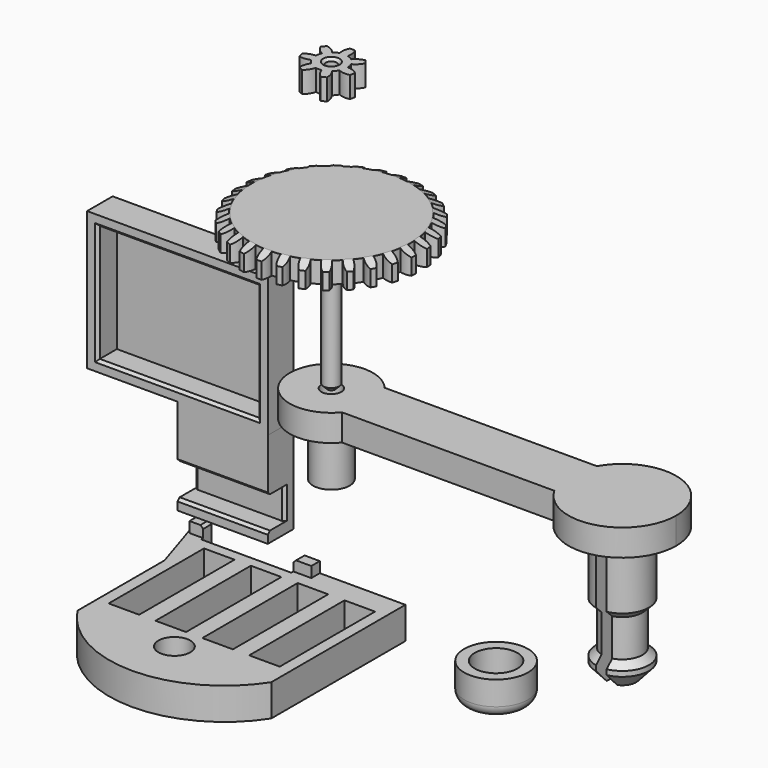
from build123d import *

# Parameters (mm, degrees)
F2_DEPTH   = 4
F3_R       = 1.05
F4_DEPTH   = 25
F5_SIZE    = 0.5
F7_DEPTH   = 4
F8_R       = 1.5
F9_DEPTH   = 25
F10_SIZE   = 0.8
F12_W      = 30
F12_H      = 22
F13_DEPTH  = 1.5
F12_W_2    = 16.9512806386
F12_H_2    = 18
F14_DEPTH  = 6
F16_W      = 5.7375021279
F16_H      = 22.3875014344
F16_R      = 3
F16_W_2    = 19.4487193614
F16_H_2    = 2
F17_DEPTH  = 6
F19_W      = 5.8088458058
F19_H      = 6
F20_DEPTH  = 25
F21_W      = 3.3711902797
F21_H      = 2
F22_DEPTH  = 2
F23_SIZE   = 0.5
F23_2_SIZE = 0.5
F26_DEPTH  = 5
F27_R      = 3.4403136116
F28_DEPTH  = 10
F29_R      = 1.35
F30_DEPTH  = 15
F30_TAPER  = -2
F31_R      = 5
F32_DEPTH  = 25
F33_W      = 2
F33_H      = 11.0666673959
F34_DEPTH  = 25
F38_R      = 6
F38_R_2    = 4
F39_DEPTH  = 6.5
F40_R      = 1.99999


# Not quite as in the source:
# - a fillet or chamfer is up to 0.001 mm smaller than in the source, because OpenCascade refuses the exact size


with BuildPart() as f2:
    # F1 (on offset) → F2 (new body)
    with BuildSketch(Plane.XY.offset(25)):
        with BuildLine():
            ThreePointArc((0.7727213217, 2.898775907), (0.8079351244, 3.9593943014), (0.5, 4.9749371855))
            ThreePointArc((0.5, 4.9749371855), (0, 5), (-0.5, 4.9749371855))
            ThreePointArc((-0.5, 4.9749371855), (-0.8079351244, 3.9593943014), (-0.7727213217, 2.898775907))
            ThreePointArc((-0.7727213217, 2.898775907), (-1.3029249894, 2.7055516185), (-1.7845704009, 2.4114950724))
            ThreePointArc((-1.7845704009, 2.4114950724), (-2.5918398057, 3.1003110845), (-3.577817614, 3.4927383413))
            ThreePointArc((-3.577817614, 3.4927383413), (-3.9091574123, 3.1174490093), (-4.2013074159, 2.7109068588))
            ThreePointArc((-4.2013074159, 2.7109068588), (-3.599318427, 1.8369728524), (-2.7481381285, 1.2032193594))
            ThreePointArc((-2.7481381285, 1.2032193594), (-2.9276458763, 0.6682160666), (-2.9980442131, 0.1083092627))
            ThreePointArc((-2.9980442131, 0.1083092627), (-4.0399064982, -0.0933696138), (-4.9614655905, -0.6195637128))
            ThreePointArc((-4.9614655905, -0.6195637128), (-4.8746395609, -1.1126046698), (-4.7389446565, -1.594491625))
            ThreePointArc((-4.7389446565, -1.594491625), (-3.6803415413, -1.6687266219), (-2.6541508727, -1.398385907))
            ThreePointArc((-2.6541508727, -1.398385907), (-2.3477897053, -1.8722998126), (-1.9539295838, -2.2764356309))
            ThreePointArc((-1.9539295838, -2.2764356309), (-2.4458411985, -3.2167410885), (-2.6090287819, -4.2653216544))
            ThreePointArc((-2.6090287819, -4.2653216544), (-2.1694186956, -4.5048443395), (-1.708059914, -4.6992053935))
            ThreePointArc((-1.708059914, -4.6992053935), (-0.9899924097, -3.9178409141), (-0.561533875, -2.9469780636))
            ThreePointArc((-0.561533875, -2.9469780636), (0, -3.002935745), (0.561533875, -2.9469780636))
            ThreePointArc((0.561533875, -2.9469780636), (0.9899924097, -3.9178409141), (1.708059914, -4.6992053935))
            ThreePointArc((1.708059914, -4.6992053935), (2.1694186956, -4.5048443395), (2.6090287819, -4.2653216544))
            ThreePointArc((2.6090287819, -4.2653216544), (2.4458411985, -3.2167410885), (1.9539295838, -2.2764356309))
            ThreePointArc((1.9539295838, -2.2764356309), (2.3477897053, -1.8722998126), (2.6541508727, -1.398385907))
            ThreePointArc((2.6541508727, -1.398385907), (3.6803415413, -1.6687266219), (4.7389446565, -1.594491625))
            ThreePointArc((4.7389446565, -1.594491625), (4.8746395609, -1.1126046698), (4.9614655905, -0.6195637128))
            ThreePointArc((4.9614655905, -0.6195637128), (4.0399064982, -0.0933696138), (2.9980442131, 0.1083092627))
            ThreePointArc((2.9980442131, 0.1083092627), (2.9276458763, 0.6682160666), (2.7481381285, 1.2032193594))
            ThreePointArc((2.7481381285, 1.2032193594), (3.599318427, 1.8369728524), (4.2013074159, 2.7109068588))
            ThreePointArc((4.2013074159, 2.7109068588), (3.9091574123, 3.1174490093), (3.577817614, 3.4927383413))
            ThreePointArc((3.577817614, 3.4927383413), (2.5918398057, 3.1003110845), (1.7845704009, 2.4114950724))
            ThreePointArc((1.7845704009, 2.4114950724), (1.3029249894, 2.7055516185), (0.7727213217, 2.898775907))
        make_face()
    extrude(amount=F2_DEPTH)

    # F3 (on offset) → F4 (cut)
    with BuildSketch(Plane.XY.offset(25)):
        Circle(F3_R)
    extrude(amount=F4_DEPTH, mode=Mode.SUBTRACT)

    # F5
    f5_edges = [f2.edges().sort_by_distance(p)[0] for p in [
        (-1.05, 0, 25),
        (-1.05, 0, 29),
    ]]
    chamfer(f5_edges, length=F5_SIZE)


with BuildPart() as f7:
    # F6 (on Top) → F7 (new body)
    with BuildSketch(Plane.XY):
        with BuildLine():
            ThreePointArc((0.77, 14.9802236298), (0.7961919909, 16.0080611466), (0.5, 16.992645468))
            ThreePointArc((0.5, 16.992645468), (0, 17), (-0.5, 16.992645468))
            ThreePointArc((-0.5, 16.992645468), (-0.7961919909, 16.0080611466), (-0.77, 14.9802236298))
            ThreePointArc((-0.77, 14.9802236298), (-1.5695471771, 14.9332438715), (-2.3613899711, 14.8129618039))
            ThreePointArc((-2.3613899711, 14.8129618039), (-2.5494697741, 15.823784226), (-3.0438958503, 16.72527124))
            ThreePointArc((-3.0438958503, 16.72527124), (-3.5344987439, 16.6285092125), (-4.0220434511, 16.5173595492))
            ThreePointArc((-4.0220434511, 16.5173595492), (-4.1070563453, 15.4927089799), (-3.8677372763, 14.4927778001))
            ThreePointArc((-3.8677372763, 14.4927778001), (-4.6400447883, 14.2805894566), (-5.3895758693, 13.9983024667))
            ThreePointArc((-5.3895758693, 13.9983024667), (-5.7837074763, 14.9479320038), (-6.4547588458, 15.7269224021))
            ThreePointArc((-6.4547588458, 15.7269224021), (-6.9145229323, 15.5302727799), (-7.3683043034, 15.3201857591))
            ThreePointArc((-7.3683043034, 15.3201857591), (-7.2384226296, 14.3002510886), (-6.7964358741, 13.3719280363))
            ThreePointArc((-6.7964358741, 13.3719280363), (-7.5077501768, 13.0038047567), (-8.18221144, 12.5718501403))
            ThreePointArc((-8.18221144, 12.5718501403), (-8.7651694084, 13.4187834248), (-9.5835179063, 14.0412315891))
            ThreePointArc((-9.5835179063, 14.0412315891), (-9.992349289, 13.7532889044), (-10.3925349007, 13.4534463368))
            ThreePointArc((-10.3925349007, 13.4534463368), (-10.0534351112, 12.4828036044), (-9.4280976113, 11.6666608518))
            ThreePointArc((-9.4280976113, 11.6666608518), (-10.0473308563, 11.1586913897), (-10.6172451081, 10.5959476364))
            ThreePointArc((-10.6172451081, 10.5959476364), (-11.3635513774, 11.3031696198), (-12.2934312475, 11.7418715784))
            ThreePointArc((-12.2934312475, 11.7418715784), (-12.6334620331, 11.3752203081), (-12.9625618539, 10.9987267529))
            ThreePointArc((-12.9625618539, 10.9987267529), (-12.4290642367, 10.1197977036), (-11.6477062419, 9.4515046052))
            ThreePointArc((-11.6477062419, 9.4515046052), (-12.147794965, 8.8258896636), (-12.5882542178, 8.1569513758))
            ThreePointArc((-12.5882542178, 8.1569513758), (-13.4652916229, 8.6935530637), (-14.4660626528, 8.9293354359))
            ThreePointArc((-14.4660626528, 8.9293354359), (-14.7224318643, 8.5), (-14.9660626528, 8.0633100321))
            ThreePointArc((-14.9660626528, 8.0633100321), (-14.2614836137, 7.3145080829), (-13.3582542178, 6.823272254))
            ThreePointArc((-13.3582542178, 6.823272254), (-13.7173421422, 6.1073542079), (-14.009096213, 5.3614571987))
            ThreePointArc((-14.009096213, 5.3614571987), (-14.9785340108, 5.7039865224), (-16.0064577042, 5.7265444871))
            ThreePointArc((-16.0064577042, 5.7265444871), (-16.167960777, 5.2532889044), (-16.3154746986, 4.7754879708))
            ThreePointArc((-16.3154746986, 4.7754879708), (-15.4706077227, 4.1895393602), (-14.4849823844, 3.8968301636))
            ThreePointArc((-14.4849823844, 3.8968301636), (-14.6873756446, 3.121898067), (-14.8176734807, 2.3316416149))
            ThreePointArc((-14.8176734807, 2.3316416149), (-15.8371425874, 2.4651283994), (-16.8472937465, 2.2734760653))
            ThreePointArc((-16.8472937465, 2.2734760653), (-16.9068722213, 1.7769838756), (-16.9518222098, 1.2789541699))
            ThreePointArc((-16.9518222098, 1.2789541699), (-16.003592038, 0.8814676637), (-14.9786473141, 0.800077896))
            ThreePointArc((-14.9786473141, 0.800077896), (-15.0155003535, 0), (-14.9786473141, -0.800077896))
            ThreePointArc((-14.9786473141, -0.800077896), (-16.003592038, -0.8814676637), (-16.9518222098, -1.2789541699))
            ThreePointArc((-16.9518222098, -1.2789541699), (-16.9068722213, -1.7769838756), (-16.8472937465, -2.2734760653))
            ThreePointArc((-16.8472937465, -2.2734760653), (-15.8371425874, -2.4651283994), (-14.8176734807, -2.3316416149))
            ThreePointArc((-14.8176734807, -2.3316416149), (-14.6873756446, -3.121898067), (-14.4849823844, -3.8968301636))
            ThreePointArc((-14.4849823844, -3.8968301636), (-15.4706077227, -4.1895393602), (-16.3154746986, -4.7754879708))
            ThreePointArc((-16.3154746986, -4.7754879708), (-16.167960777, -5.2532889044), (-16.0064577042, -5.7265444871))
            ThreePointArc((-16.0064577042, -5.7265444871), (-14.9785340108, -5.7039865224), (-14.009096213, -5.3614571987))
            ThreePointArc((-14.009096213, -5.3614571987), (-13.7173421422, -6.1073542079), (-13.3582542178, -6.823272254))
            ThreePointArc((-13.3582542178, -6.823272254), (-14.2614836137, -7.3145080829), (-14.9660626528, -8.0633100321))
            ThreePointArc((-14.9660626528, -8.0633100321), (-14.7224318643, -8.5), (-14.4660626528, -8.9293354359))
            ThreePointArc((-14.4660626528, -8.9293354359), (-13.4652916229, -8.6935530637), (-12.5882542178, -8.1569513758))
            ThreePointArc((-12.5882542178, -8.1569513758), (-12.147794965, -8.8258896636), (-11.6477062419, -9.4515046052))
            ThreePointArc((-11.6477062419, -9.4515046052), (-12.4290642367, -10.1197977036), (-12.9625618539, -10.9987267529))
            ThreePointArc((-12.9625618539, -10.9987267529), (-12.6334620331, -11.3752203081), (-12.2934312475, -11.7418715784))
            ThreePointArc((-12.2934312475, -11.7418715784), (-11.3635513774, -11.3031696198), (-10.6172451081, -10.5959476364))
            ThreePointArc((-10.6172451081, -10.5959476364), (-10.0473308563, -11.1586913897), (-9.4280976113, -11.6666608518))
            ThreePointArc((-9.4280976113, -11.6666608518), (-10.0534351112, -12.4828036044), (-10.3925349007, -13.4534463368))
            ThreePointArc((-10.3925349007, -13.4534463368), (-9.992349289, -13.7532889044), (-9.5835179063, -14.0412315891))
            ThreePointArc((-9.5835179063, -14.0412315891), (-8.7651694084, -13.4187834248), (-8.18221144, -12.5718501403))
            ThreePointArc((-8.18221144, -12.5718501403), (-7.5077501768, -13.0038047567), (-6.7964358741, -13.3719280363))
            ThreePointArc((-6.7964358741, -13.3719280363), (-7.2384226296, -14.3002510886), (-7.3683043034, -15.3201857591))
            ThreePointArc((-7.3683043034, -15.3201857591), (-6.9145229323, -15.5302727799), (-6.4547588458, -15.7269224021))
            ThreePointArc((-6.4547588458, -15.7269224021), (-5.7837074763, -14.9479320038), (-5.3895758693, -13.9983024667))
            ThreePointArc((-5.3895758693, -13.9983024667), (-4.6400447883, -14.2805894566), (-3.8677372763, -14.4927778001))
            ThreePointArc((-3.8677372763, -14.4927778001), (-4.1070563453, -15.4927089799), (-4.0220434511, -16.5173595492))
            ThreePointArc((-4.0220434511, -16.5173595492), (-3.5344987439, -16.6285092125), (-3.0438958503, -16.72527124))
            ThreePointArc((-3.0438958503, -16.72527124), (-2.5494697741, -15.823784226), (-2.3613899711, -14.8129618039))
            ThreePointArc((-2.3613899711, -14.8129618039), (-1.5695471771, -14.9332438715), (-0.77, -14.9802236298))
            ThreePointArc((-0.77, -14.9802236298), (-0.7961919909, -16.0080611466), (-0.5, -16.992645468))
            ThreePointArc((-0.5, -16.992645468), (0, -17), (0.5, -16.992645468))
            ThreePointArc((0.5, -16.992645468), (0.7961919909, -16.0080611466), (0.77, -14.9802236298))
            ThreePointArc((0.77, -14.9802236298), (1.5695471771, -14.9332438715), (2.3613899711, -14.8129618039))
            ThreePointArc((2.3613899711, -14.8129618039), (2.5494697741, -15.823784226), (3.0438958503, -16.72527124))
            ThreePointArc((3.0438958503, -16.72527124), (3.5344987439, -16.6285092125), (4.0220434511, -16.5173595492))
            ThreePointArc((4.0220434511, -16.5173595492), (4.1070563453, -15.4927089799), (3.8677372763, -14.4927778001))
            ThreePointArc((3.8677372763, -14.4927778001), (4.6400447883, -14.2805894566), (5.3895758693, -13.9983024667))
            ThreePointArc((5.3895758693, -13.9983024667), (5.7837074763, -14.9479320038), (6.4547588458, -15.7269224021))
            ThreePointArc((6.4547588458, -15.7269224021), (6.9145229323, -15.5302727799), (7.3683043034, -15.3201857591))
            ThreePointArc((7.3683043034, -15.3201857591), (7.2384226296, -14.3002510886), (6.7964358741, -13.3719280363))
            ThreePointArc((6.7964358741, -13.3719280363), (7.5077501768, -13.0038047567), (8.18221144, -12.5718501403))
            ThreePointArc((8.18221144, -12.5718501403), (8.7651694084, -13.4187834248), (9.5835179063, -14.0412315891))
            ThreePointArc((9.5835179063, -14.0412315891), (9.992349289, -13.7532889044), (10.3925349007, -13.4534463368))
            ThreePointArc((10.3925349007, -13.4534463368), (10.0534351112, -12.4828036044), (9.4280976113, -11.6666608518))
            ThreePointArc((9.4280976113, -11.6666608518), (10.0473308563, -11.1586913897), (10.6172451081, -10.5959476364))
            ThreePointArc((10.6172451081, -10.5959476364), (11.3635513774, -11.3031696198), (12.2934312475, -11.7418715784))
            ThreePointArc((12.2934312475, -11.7418715784), (12.6334620331, -11.3752203081), (12.9625618539, -10.9987267529))
            ThreePointArc((12.9625618539, -10.9987267529), (12.4290642367, -10.1197977036), (11.6477062419, -9.4515046052))
            ThreePointArc((11.6477062419, -9.4515046052), (12.147794965, -8.8258896636), (12.5882542178, -8.1569513758))
            ThreePointArc((12.5882542178, -8.1569513758), (13.4652916229, -8.6935530637), (14.4660626528, -8.9293354359))
            ThreePointArc((14.4660626528, -8.9293354359), (14.7224318643, -8.5), (14.9660626528, -8.0633100321))
            ThreePointArc((14.9660626528, -8.0633100321), (14.2614836137, -7.3145080829), (13.3582542178, -6.823272254))
            ThreePointArc((13.3582542178, -6.823272254), (13.7173421422, -6.1073542079), (14.009096213, -5.3614571987))
            ThreePointArc((14.009096213, -5.3614571987), (14.9785340108, -5.7039865224), (16.0064577042, -5.7265444871))
            ThreePointArc((16.0064577042, -5.7265444871), (16.167960777, -5.2532889044), (16.3154746986, -4.7754879708))
            ThreePointArc((16.3154746986, -4.7754879708), (15.4706077227, -4.1895393602), (14.4849823844, -3.8968301636))
            ThreePointArc((14.4849823844, -3.8968301636), (14.6873756446, -3.121898067), (14.8176734807, -2.3316416149))
            ThreePointArc((14.8176734807, -2.3316416149), (15.8371425874, -2.4651283994), (16.8472937465, -2.2734760653))
            ThreePointArc((16.8472937465, -2.2734760653), (16.9068722213, -1.7769838756), (16.9518222098, -1.2789541699))
            ThreePointArc((16.9518222098, -1.2789541699), (16.003592038, -0.8814676637), (14.9786473141, -0.800077896))
            ThreePointArc((14.9786473141, -0.800077896), (15.0155003535, 0), (14.9786473141, 0.800077896))
            ThreePointArc((14.9786473141, 0.800077896), (16.003592038, 0.8814676637), (16.9518222098, 1.2789541699))
            ThreePointArc((16.9518222098, 1.2789541699), (16.9068722213, 1.7769838756), (16.8472937465, 2.2734760653))
            ThreePointArc((16.8472937465, 2.2734760653), (15.8371425874, 2.4651283994), (14.8176734807, 2.3316416149))
            ThreePointArc((14.8176734807, 2.3316416149), (14.6873756446, 3.121898067), (14.4849823844, 3.8968301636))
            ThreePointArc((14.4849823844, 3.8968301636), (15.4706077227, 4.1895393602), (16.3154746986, 4.7754879708))
            ThreePointArc((16.3154746986, 4.7754879708), (16.167960777, 5.2532889044), (16.0064577042, 5.7265444871))
            ThreePointArc((16.0064577042, 5.7265444871), (14.9785340108, 5.7039865224), (14.009096213, 5.3614571987))
            ThreePointArc((14.009096213, 5.3614571987), (13.7173421422, 6.1073542079), (13.3582542178, 6.823272254))
            ThreePointArc((13.3582542178, 6.823272254), (14.2614836137, 7.3145080829), (14.9660626528, 8.0633100321))
            ThreePointArc((14.9660626528, 8.0633100321), (14.7224318643, 8.5), (14.4660626528, 8.9293354359))
            ThreePointArc((14.4660626528, 8.9293354359), (13.4652916229, 8.6935530637), (12.5882542178, 8.1569513758))
            ThreePointArc((12.5882542178, 8.1569513758), (12.147794965, 8.8258896636), (11.6477062419, 9.4515046052))
            ThreePointArc((11.6477062419, 9.4515046052), (12.4290642367, 10.1197977036), (12.9625618539, 10.9987267529))
            ThreePointArc((12.9625618539, 10.9987267529), (12.6334620331, 11.3752203081), (12.2934312475, 11.7418715784))
            ThreePointArc((12.2934312475, 11.7418715784), (11.3635513774, 11.3031696198), (10.6172451081, 10.5959476364))
            ThreePointArc((10.6172451081, 10.5959476364), (10.0473308563, 11.1586913897), (9.4280976113, 11.6666608518))
            ThreePointArc((9.4280976113, 11.6666608518), (10.0534351112, 12.4828036044), (10.3925349007, 13.4534463368))
            ThreePointArc((10.3925349007, 13.4534463368), (9.992349289, 13.7532889044), (9.5835179063, 14.0412315891))
            ThreePointArc((9.5835179063, 14.0412315891), (8.7651694084, 13.4187834248), (8.18221144, 12.5718501403))
            ThreePointArc((8.18221144, 12.5718501403), (7.5077501768, 13.0038047567), (6.7964358741, 13.3719280363))
            ThreePointArc((6.7964358741, 13.3719280363), (7.2384226296, 14.3002510886), (7.3683043034, 15.3201857591))
            ThreePointArc((7.3683043034, 15.3201857591), (6.9145229323, 15.5302727799), (6.4547588458, 15.7269224021))
            ThreePointArc((6.4547588458, 15.7269224021), (5.7837074763, 14.9479320038), (5.3895758693, 13.9983024667))
            ThreePointArc((5.3895758693, 13.9983024667), (4.6400447883, 14.2805894566), (3.8677372763, 14.4927778001))
            ThreePointArc((3.8677372763, 14.4927778001), (4.1070563453, 15.4927089799), (4.0220434511, 16.5173595492))
            ThreePointArc((4.0220434511, 16.5173595492), (3.5344987439, 16.6285092125), (3.0438958503, 16.72527124))
            ThreePointArc((3.0438958503, 16.72527124), (2.5494697741, 15.823784226), (2.3613899711, 14.8129618039))
            ThreePointArc((2.3613899711, 14.8129618039), (1.5695471771, 14.9332438715), (0.77, 14.9802236298))
        make_face()
    extrude(amount=F7_DEPTH)

    # F8 (on Top) → F9 (join)
    with BuildSketch(Plane.XY):
        Circle(F8_R)
    extrude(amount=-F9_DEPTH)

    # F10
    f10_edges = [f7.edges().sort_by_distance(p)[0] for p in [
        (-1.5, 0, 0),
        (-1.5, 0, -25),
    ]]
    chamfer(f10_edges, length=F10_SIZE)

    # F41 (on Right) → F42 (revolve, cut)
    with BuildSketch(Plane.YZ):
        Polygon((-17.2905419022, 2.8945491649), (-13.9582687989, 4.4342144392), (-17.2905419022, 4.5154177751), align=None)
    revolve(axis=Axis((0, 0, 0), (0, 0, 1)), mode=Mode.SUBTRACT)


with BuildPart() as f13:
    # F12 (on offset) → F13 (new body)
    with BuildSketch(Plane.XZ.offset(-25)):
        Polygon((-27.0875040293, -23.2919594112), (-61.0875040293, -23.2919594112), (-61.0875040293, -49.2919594112), (-44.0875040293, -49.2919594112), (-27.1362233907, -49.2919594112), (-27.0875040293, -49.2919594112), align=None)
        with Locations((-44.0875040293, -36.2919594112)):
            Rectangle(F12_W, F12_H, mode=Mode.SUBTRACT)
        with Locations((-44.0875040293, -36.2919594112)):
            Rectangle(F12_W, F12_H)
    extrude(amount=F13_DEPTH)

    # F12 (on offset) → F14 (join)
    with BuildSketch(Plane.XZ.offset(-25)):
        Polygon((-27.0875040293, -23.2919594112), (-61.0875040293, -23.2919594112), (-61.0875040293, -49.2919594112), (-44.0875040293, -49.2919594112), (-27.1362233907, -49.2919594112), (-27.0875040293, -49.2919594112), align=None)
        with Locations((-44.0875040293, -36.2919594112)):
            Rectangle(F12_W, F12_H, mode=Mode.SUBTRACT)
        with Locations((-35.61186371, -58.2919594112)):
            Rectangle(F12_W_2, F12_H_2)
    extrude(amount=F14_DEPTH)

    # F19 (on offset) → F20 (cut)
    with BuildSketch(Plane(origin=(-44.0875040293, 0, 0), x_dir=(0, -1, 0), z_dir=(-1, 0, 0))):
        with Locations((-20.0955770971, -62.2919594112)):
            Rectangle(F19_W, F19_H)
    extrude(amount=-F20_DEPTH, mode=Mode.SUBTRACT)

    # F23
    f23_edges = [f13.edges().sort_by_distance(p)[0] for p in [
        (-35.611864, 19, -65.291959),
        (-35.611864, 19, -59.291959),
        (-44.087504, 23, -62.291959),
        (-27.136223, 23, -62.291959),
        (-29.087504, 19, -36.291959),
        (-44.087504, 19, -25.291959),
        (-44.087504, 19, -47.291959),
        (-59.087504, 19, -36.291959),
    ]]
    chamfer(f23_edges, length=F23_SIZE)


with BuildPart() as f17:
    # F16 (on offset) → F17 (new body)
    with BuildSketch(Plane(origin=(0, 0, -74.2919594112), x_dir=(1, 0, 0), z_dir=(0, 0, -1))):
        with BuildLine():
            Line((-44.0875040293, -15.9287359565), (-44.0875040293, -25))
            Line((-44.0875040293, -25), (-27.1362233907, -25))
            Line((-27.1362233907, -25), (-7.6875040293, -25))
            Line((-7.6875040293, -25), (-7.6875040293, 4.5))
            ThreePointArc((-7.6875040293, 4.5), (-25.8875040293, 14.4115268461), (-44.0875040293, 4.5))
            Line((-44.0875040293, 4.5), (-44.0875040293, -15.9287359565))
        make_face()
        with Locations((-39.077790454, -11.3334820489)):
            Rectangle(F16_W, F16_H, mode=Mode.SUBTRACT)
        with Locations((-30.277790454, -11.3334820489)):
            Rectangle(F16_W, F16_H, mode=Mode.SUBTRACT)
        with Locations((-21.477790454, -11.3334820489)):
            Rectangle(F16_W, F16_H, mode=Mode.SUBTRACT)
        with Locations((-12.677790454, -11.3334820489)):
            Rectangle(F16_W, F16_H, mode=Mode.SUBTRACT)
        with Locations((-25.8875040293, 4.5)):
            Circle(F16_R, mode=Mode.SUBTRACT)
        Polygon((-44.1308841109, -27), (-44.0875040293, -25), (-44.0875040293, -15.9287359565), (-47.6132445037, -27), align=None)
        with Locations((-17.41186371, -26)):
            Rectangle(F16_W_2, F16_H_2)
    extrude(amount=F17_DEPTH)

    # F21 (on offset) → F22 (join)
    with BuildSketch(Plane(origin=(0, 0, -74.2919594112), x_dir=(1, 0, 0), z_dir=(0, 0, -1))):
        Polygon((-44.0875040293, -25), (-46.6469936073, -25), (-46.6469936073, -27), (-44.1308841109, -27), align=None)
        with Locations((-25.4506282508, -26)):
            Rectangle(F21_W, F21_H)
    extrude(amount=-F22_DEPTH)

    # F23#2
    f23_2_edges = [f17.edges().sort_by_distance(p)[0] for p in [
        (-27.136223, 26, -72.291959),
        (-44.109194, 26, -72.291959),
        (-35.611864, 25, -80.291959),
        (-35.611864, 25, -74.291959),
    ]]
    chamfer(f23_2_edges, length=F23_2_SIZE)


with BuildPart() as f26:
    # F25 (on offset) → F26 (new body)
    with BuildSketch(Plane.XY.offset(-30)):
        with BuildLine():
            ThreePointArc((6.0099373656, -4.9977370421), (7.3509534431, -2.657104845), (7.8164392584, 0))
            ThreePointArc((7.8164392584, 0), (7.3509534431, 2.657104845), (6.0099373656, 4.9977370421))
            ThreePointArc((6.0099373656, 4.9977370421), (-7.8164392584, 0), (6.0099373656, -4.9977370421))
        make_face()
        with BuildLine():
            ThreePointArc((6.0099373656, 4.9977370421), (7.3509534431, 2.657104845), (7.8164392584, 0))
            ThreePointArc((7.8164392584, 0), (7.3509534431, -2.657104845), (6.0099373656, -4.9977370421))
            Line((6.0099373656, -4.9977370421), (45.8839294917, -4.9977370421))
            ThreePointArc((45.8839294917, -4.9977370421), (44.5624056209, 0), (45.8839294917, 4.9977370421))
            Line((45.8839294917, 4.9977370421), (6.0099373656, 4.9977370421))
        make_face()
        with BuildLine():
            ThreePointArc((64.7843641292, 0), (57.2581382909, 9.7750166883), (45.8839294917, 4.9977370421))
            ThreePointArc((45.8839294917, 4.9977370421), (44.5624056209, 0), (45.8839294917, -4.9977370421))
            ThreePointArc((45.8839294917, -4.9977370421), (57.2581382909, -9.7750166883), (64.7843641292, 0))
        make_face()
    extrude(amount=F26_DEPTH)

    # F27 (on face) → F28 (join)
    with BuildSketch(Plane(origin=(0, 0, -30), x_dir=(1, 0, 0), z_dir=(0, 0, -1))):
        Circle(F27_R)
    extrude(amount=F28_DEPTH)

    # F29 (on face) → F30 (cut)
    with BuildSketch(Plane(origin=(0, 0, -40), x_dir=(1, 0, 0), z_dir=(0, 0, -1))):
        Circle(F29_R)
    extrude(amount=-F30_DEPTH, taper=F30_TAPER, mode=Mode.SUBTRACT)

    # F31 (on face) → F32 (join)
    with BuildSketch(Plane(origin=(0, 0, -30), x_dir=(1, 0, 0), z_dir=(0, 0, -1))):
        with Locations((54.6733848751, 0)):
            Circle(F31_R)
    extrude(amount=F32_DEPTH)

    # F33 (on face) → F34 (cut)
    with BuildSketch(Plane(origin=(0, 0, -55), x_dir=(1, 0, 0), z_dir=(0, 0, -1))):
        with Locations((54.6514354646, -0.1308538485)):
            Rectangle(F33_W, F33_H)
    extrude(amount=-F34_DEPTH, mode=Mode.SUBTRACT)

    # F35 (on Front) → F36 (revolve, cut)
    with BuildSketch(Plane.XZ):
        Polygon((60.0431378339, -51.7530592644), (60.0431378339, -41.5070942368), (58.4201553201, -43.1300767506), (58.4201553201, -50.1300767506), align=None)
        Polygon((59.9594203222, -52.0358361038), (56.4293397813, -55.9424627704), (59.9594203222, -55.9424627704), align=None)
    revolve(axis=Axis((54.6733848751, 0, -30), (0, 0, 1)), mode=Mode.SUBTRACT)


with BuildPart() as f39:
    # F38 (on offset) → F39 (new body)
    with BuildSketch(Plane(origin=(0, 0, -60), x_dir=(1, 0, 0), z_dir=(0, 0, -1))):
        with Locations((30.9499785999, 0)):
            Circle(F38_R)
        with Locations((30.9499785999, 0)):
            Circle(F38_R_2, mode=Mode.SUBTRACT)
    extrude(amount=F39_DEPTH)

    # F40 (radius 2 in the source; OpenCascade refuses exactly that, so slightly less here)
    f40_edges = [f39.edges().sort_by_distance(p)[0] for p in [
        (24.949979, 0, -66.5),
    ]]
    fillet(f40_edges, radius=F40_R)


solid = Compound([f2.part, f7.part, f13.part, f17.part, f26.part, f39.part])
